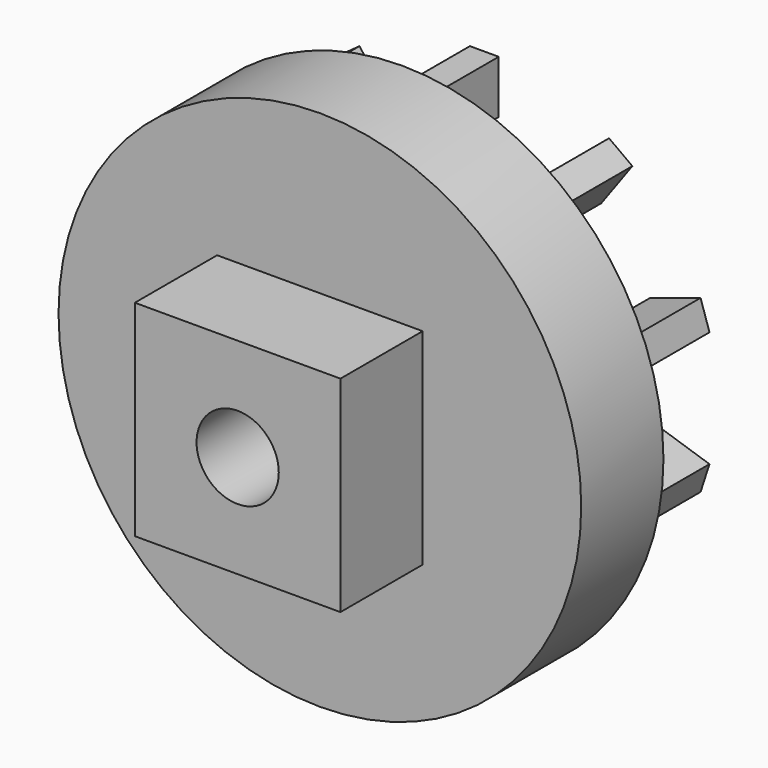
from build123d import *
from build123d import SkipClean  # not in build123d's __all__

# Parameters (mm, degrees)
F0_R     = 63.5754098613
F1_DEPTH = 25
F2_R     = 10
F3_DEPTH = 25.001
F4_W     = 50
F4_H     = 50
F4_R     = 10
F5_DEPTH = 25
F6_W     = 7.0136869326
F6_H     = 12.901866436
F7_DEPTH = 25
F8_COUNT = 10


# Not quite as in the source:
# - after a boolean that leaves OpenCascade's solid faulty, fix() repairs it


with BuildPart() as f1:
    # F0 (on Front) → F1 (new body)
    with BuildSketch(Plane.XZ):
        Circle(F0_R)
    extrude(amount=F1_DEPTH)

    # F2 (on face) → F3 (cut, through all)
    with BuildSketch(Plane(origin=(0, 0, 0), x_dir=(-1, 0, 0), z_dir=(0, 1, 0))):
        Circle(F2_R)
    extrude(amount=-F3_DEPTH, mode=Mode.SUBTRACT)

    # F4 (on face) → F5 (join)
    with BuildSketch(Plane.XZ.offset(25)):
        Rectangle(F4_W, F4_H)
        Circle(F4_R, mode=Mode.SUBTRACT)
    with SkipClean():  # cleaning this boolean's faces spoils the solid; the shape is the same uncleaned
        extrude(amount=F5_DEPTH)

    # F6 (on face) → F7 (join)
    with BuildSketch(Plane(origin=(0, 0, 0), x_dir=(-1, 0, 0), z_dir=(0, 1, 0))):
        with Locations((0, -50)):
            Rectangle(F6_W, F6_H)
    f7 = extrude(amount=F7_DEPTH)

    add(f1.part.fix(), mode=Mode.REPLACE)

    # F8: F7 ×10 about axis
    f8_axis = Axis((0, 0, 0), (0, -1, 0))
    for i in range(1, F8_COUNT):
        add(f7.rotate(f8_axis, i * 360 / F8_COUNT), clean=False)


solid = f1.part
